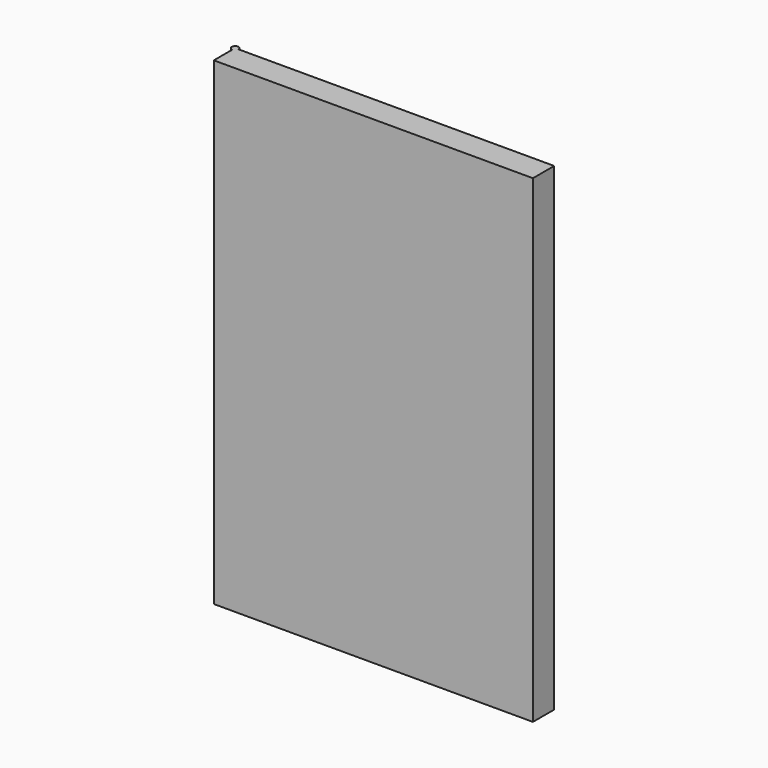
from build123d import *

# Parameters (mm, degrees)
F0_W     = 304.8
F0_H     = 457.2
F2_DEPTH = 25.4
F3_T     = -6.35
F4_W     = 3.175
F4_H     = 25.4


# Not quite as in the source:
# - the program builds the solid bodies; features that only make, move or delete a surface that nothing else refers to are left out


with BuildPart() as f2:
    # F0 (on Front) → F2 (new body)
    with BuildSketch(Plane.XZ):
        with Locations((152.4, -228.6)):
            Rectangle(F0_W, F0_H)
    extrude(amount=F2_DEPTH)

    # F3
    f3_openings = [f2.faces().sort_by_distance(p)[0] for p in [
        (152.4, 0, -228.6),
    ]]
    offset(amount=F3_T, openings=f3_openings)

    # F4 (on Right) → F5 (revolve)
    with BuildSketch(Plane.YZ):
        with Locations((1.5875, -12.7)):
            Rectangle(F4_W, F4_H)
    revolve(axis=Axis((0, 0, 39.7453531623), (0, 0, 1)))


solid = f2.part
